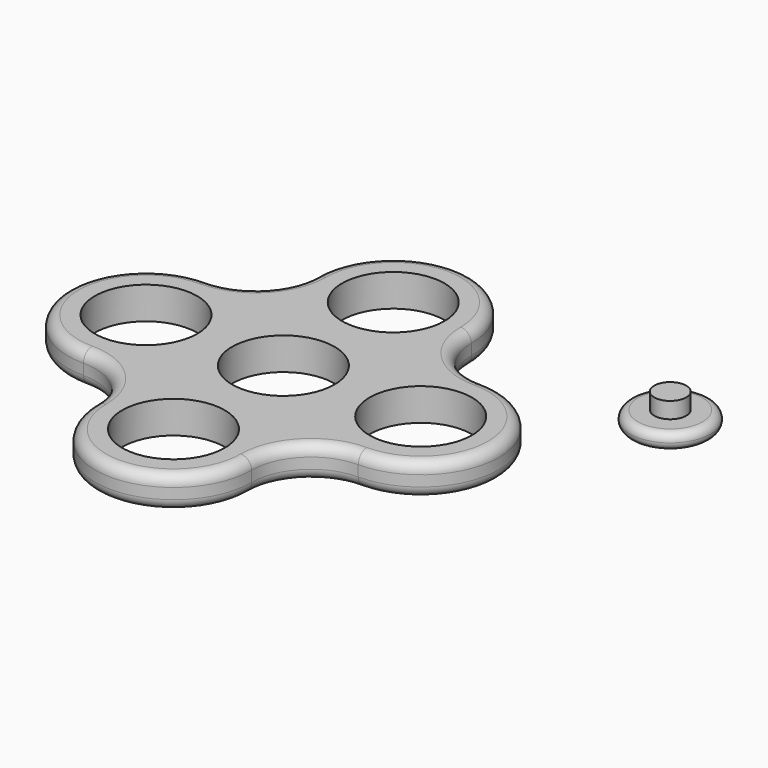
from build123d import *

# Parameters (mm, degrees)
F0_R     = 9.5
F1_DEPTH = 6
F2_R     = 2
F3_R     = 2.965
F4_DEPTH = 6
F3_R_2   = 7.5
F5_DEPTH = 3
F6_R     = 1.49999


# Not quite as in the source:
# - a fillet or chamfer is up to 0.001 mm smaller than in the source, because OpenCascade refuses the exact size


with BuildPart() as f1:
    # F0 (on Top) → F1 (new body)
    with BuildSketch(Plane.XY):
        with BuildLine():
            ThreePointArc((25.5, 14.5), (17.7218254069, 17.7218254069), (14.5, 25.5))
            ThreePointArc((14.5, 25.5), (0, 40), (-14.5, 25.5))
            ThreePointArc((-14.5, 25.5), (-17.7218254069, 17.7218254069), (-25.5, 14.5))
            ThreePointArc((-25.5, 14.5), (-40, 0), (-25.5, -14.5))
            ThreePointArc((-25.5, -14.5), (-17.7218254069, -17.7218254069), (-14.5, -25.5))
            ThreePointArc((-14.5, -25.5), (0, -40), (14.5, -25.5))
            ThreePointArc((14.5, -25.5), (17.7218254069, -17.7218254069), (25.5, -14.5))
            ThreePointArc((25.5, -14.5), (40, 0), (25.5, 14.5))
        make_face()
        with Locations((0, -25.5)):
            Circle(F0_R, mode=Mode.SUBTRACT)
        with Locations((-25.5, 0)):
            Circle(F0_R, mode=Mode.SUBTRACT)
        Circle(F0_R, mode=Mode.SUBTRACT)
        with Locations((25.5, 0)):
            Circle(F0_R, mode=Mode.SUBTRACT)
        with Locations((0, 25.5)):
            Circle(F0_R, mode=Mode.SUBTRACT)
    extrude(amount=F1_DEPTH)

    # F2
    f2_edges = [f1.edges().sort_by_distance(p)[0] for p in [
        (-40, 0, 6),
        (-17.721825, -17.721825, 6),
        (0, -40, 6),
        (17.721825, -17.721825, 6),
        (40, 0, 6),
        (17.721825, 17.721825, 6),
        (0, -40, 0),
        (-17.721825, -17.721825, 0),
        (-40, 0, 0),
        (17.721825, -17.721825, 0),
        (40, 0, 0),
        (17.721825, 17.721825, 0),
        (0, 40, 0),
        (0, 40, 6),
        (-17.721825, 17.721825, 6),
        (-17.721825, 17.721825, 0),
    ]]
    fillet(f2_edges, radius=F2_R)


with BuildPart() as f4:
    # F3 (on Top) → F4 (new body)
    with BuildSketch(Plane.XY):
        with Locations((48.8648079336, 28.6977495998)):
            Circle(F3_R)
    extrude(amount=F4_DEPTH)

    # F3 (on Top) → F5 (join)
    with BuildSketch(Plane.XY):
        with Locations((48.8648079336, 28.6977495998)):
            Circle(F3_R_2)
        with Locations((48.8648079336, 28.6977495998)):
            Circle(F3_R, mode=Mode.SUBTRACT)
    extrude(amount=F5_DEPTH)

    # F6 (radius 1.5 in the source; OpenCascade refuses exactly that, so slightly less here)
    f6_edges = [f4.edges().sort_by_distance(p)[0] for p in [
        (41.364808, 28.69775, 3),
        (41.364808, 28.69775, 0),
    ]]
    fillet(f6_edges, radius=F6_R)


solid = Compound([f1.part, f4.part])
